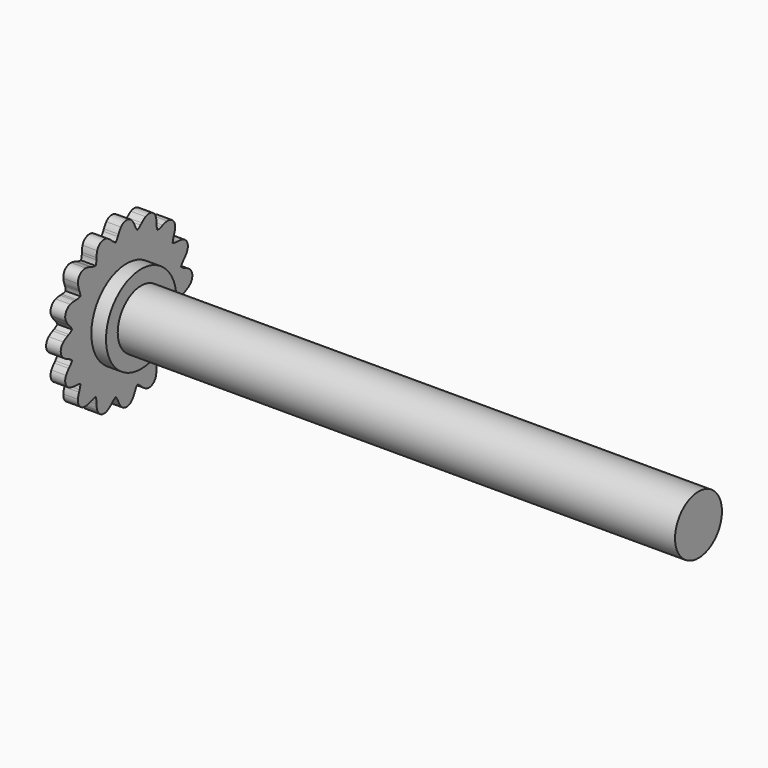
from build123d import *

# Parameters (mm, degrees)
F0_W     = 12.7
F0_H     = 12.7
F0_H_2   = 38.1
F2_R     = 25.4
F3_DEPTH = 508
F6_DEPTH = 508.001


# Not quite as in the source:
# - ends of sketch curves that miss each other by under 0.0002 mm in the source are joined


with BuildPart() as f1:
    # F0 (on Front) → F1 (revolve)
    with BuildSketch(Plane.XZ):
        with Locations((6.35, 31.75)):
            Rectangle(F0_W, F0_H)
        with Locations((19.05, 31.75)):
            Rectangle(F0_W, F0_H)
        with Locations((6.35, 57.15)):
            Rectangle(F0_W, F0_H_2)
        with Locations((19.05, -31.75)):
            Rectangle(F0_W, F0_H)
        with Locations((6.35, -31.75)):
            Rectangle(F0_W, F0_H)
        with Locations((6.35, -57.15)):
            Rectangle(F0_W, F0_H_2)
    revolve(axis=Axis((27.5155087221, 0, 0), (1, 0, 0)))


with BuildPart() as f3:
    # F2 (on face) → F3 (new body)
    with BuildSketch(Plane(origin=(0, 0, 0), x_dir=(0, -1, 0), z_dir=(-1, 0, 0))):
        Circle(F2_R)
    extrude(amount=-F3_DEPTH)

    # F4: union F1
    add(f1.part)

    # F5 (on face) → F6 (intersect, through all)
    with BuildSketch(Plane(origin=(0, 0, 0), x_dir=(0, -1, 0), z_dir=(-1, 0, 0))):
        with BuildLine():
            Line((9.3960515124, 62.4303196078), (8.6946709677, 63.9873266813))
            ThreePointArc((8.6946709677, 63.9873266813), (7.49940788, 66.2471696631), (6.0285111261, 68.338104117))
            ThreePointArc((6.0285111261, 68.338104117), (1.0289e-06, 71.2297171366), (-6.0285090682, 68.338104117))
            ThreePointArc((-6.0285090682, 68.338104117), (-7.4994058221, 66.2471696631), (-8.6946689099, 63.9873266813))
            Line((-8.6946689099, 63.9873266813), (-9.3960494545, 62.4303196078))
            ThreePointArc((-9.3960494545, 62.4303196078), (-10.4157598129, 60.5868350182), (-11.7228009421, 58.9345977067))
            ThreePointArc((-11.7228009421, 58.9345977067), (-13.5626685785, 59.9608761858), (-15.2102293125, 61.2738077372))
            Line((-15.2102293125, 61.2738077372), (-16.4540612533, 62.4438879902))
            ThreePointArc((-16.4540612533, 62.4438879902), (-18.4231448249, 64.0743032868), (-20.5822422039, 65.4431870141))
            ThreePointArc((-20.5822422039, 65.4431870141), (-27.2584316896, 65.8076781628), (-31.7214763845, 60.8291651421))
            ThreePointArc((-31.7214763845, 60.8291651421), (-32.2802418162, 58.3345057778), (-32.5197164501, 55.7892757193))
            Line((-32.5197164501, 55.7892757193), (-32.5718667687, 54.0823820379))
            ThreePointArc((-32.5718667687, 54.0823820379), (-32.8084852876, 51.9889980971), (-33.3837499896, 49.9623468766))
            ThreePointArc((-33.3837499896, 49.9623468766), (-35.4763058123, 50.2064176959), (-37.5008906056, 50.7889140871))
            Line((-37.5008906056, 50.7889140871), (-39.0978118049, 51.3939334078))
            ThreePointArc((-39.0978118049, 51.3939334078), (-41.5409407364, 52.14670507), (-44.0595357369, 52.5851379323))
            ThreePointArc((-44.0595357369, 52.5851379323), (-50.3670152817, 50.3670167368), (-52.5851364772, 44.059537192))
            ThreePointArc((-52.5851364772, 44.059537192), (-52.1467036149, 41.5409421915), (-51.3939319527, 39.09781326))
            Line((-51.3939319527, 39.09781326), (-50.788912632, 37.5008920607))
            ThreePointArc((-50.788912632, 37.5008920607), (-50.2064162869, 35.4763074971), (-49.9623257256, 33.3837816443))
            ThreePointArc((-49.9623257256, 33.3837816443), (-51.9889970797, 32.8084872341), (-54.0823812504, 32.5718686699))
            Line((-54.0823812504, 32.5718686699), (-55.7892749318, 32.5197183513))
            ThreePointArc((-55.7892749318, 32.5197183513), (-58.3345049903, 32.2802437174), (-60.8291643546, 31.7214782857))
            ThreePointArc((-60.8291643546, 31.7214782857), (-65.8076773753, 27.2584335908), (-65.4431862266, 20.5822441051))
            ThreePointArc((-65.4431862266, 20.5822441051), (-64.0743024993, 18.4231467261), (-62.4438872027, 16.4540631545))
            Line((-62.4438872027, 16.4540631545), (-61.2738069497, 15.2102312137))
            ThreePointArc((-61.2738069497, 15.2102312137), (-59.9608755289, 13.5626706742), (-58.9345902795, 11.7228382814))
            ThreePointArc((-58.9345902795, 11.7228382814), (-60.5868348232, 10.4157620005), (-62.4303196078, 9.3960515124))
            Line((-62.4303196078, 9.3960515124), (-63.9873266813, 8.6946709677))
            ThreePointArc((-63.9873266813, 8.6946709677), (-66.2471696631, 7.49940788), (-68.338104117, 6.0285111261))
            ThreePointArc((-68.338104117, 6.0285111261), (-71.2297171366, 1.0289e-06), (-68.338104117, -6.0285090682))
            ThreePointArc((-68.338104117, -6.0285090682), (-66.2471696631, -7.4994058221), (-63.9873266813, -8.6946689099))
            Line((-63.9873266813, -8.6946689099), (-62.4303196078, -9.3960494545))
            ThreePointArc((-62.4303196078, -9.3960494545), (-60.5868350182, -10.4157598129), (-58.9345977067, -11.7228009421))
            ThreePointArc((-58.9345977067, -11.7228009421), (-59.9608761858, -13.5626685785), (-61.2738077372, -15.2102293125))
            Line((-61.2738077372, -15.2102293125), (-62.4438879902, -16.4540612533))
            ThreePointArc((-62.4438879902, -16.4540612533), (-64.0743032868, -18.4231448249), (-65.4431870141, -20.5822422039))
            ThreePointArc((-65.4431870141, -20.5822422039), (-65.8076781628, -27.2584316896), (-60.8291651421, -31.7214763845))
            ThreePointArc((-60.8291651421, -31.7214763845), (-58.3345057778, -32.2802418162), (-55.7892757193, -32.5197164501))
            Line((-55.7892757193, -32.5197164501), (-54.0823820379, -32.5718667687))
            ThreePointArc((-54.0823820379, -32.5718667687), (-51.9889980971, -32.8084852876), (-49.9623468766, -33.3837499896))
            ThreePointArc((-49.9623468766, -33.3837499896), (-50.2064176959, -35.4763058123), (-50.7889140871, -37.5008906056))
            Line((-50.7889140871, -37.5008906056), (-51.3939334078, -39.0978118049))
            ThreePointArc((-51.3939334078, -39.0978118049), (-52.14670507, -41.5409407364), (-52.5851379323, -44.0595357369))
            ThreePointArc((-52.5851379323, -44.0595357369), (-50.3670167368, -50.3670152817), (-44.059537192, -52.5851364772))
            ThreePointArc((-44.059537192, -52.5851364772), (-41.5409421915, -52.1467036149), (-39.09781326, -51.3939319527))
            Line((-39.09781326, -51.3939319527), (-37.5008920607, -50.788912632))
            ThreePointArc((-37.5008920607, -50.788912632), (-35.4763074971, -50.2064162869), (-33.3837816443, -49.9623257256))
            ThreePointArc((-33.3837816443, -49.9623257256), (-32.8084872341, -51.9889970797), (-32.5718686699, -54.0823812504))
            Line((-32.5718686699, -54.0823812504), (-32.5197183513, -55.7892749318))
            ThreePointArc((-32.5197183513, -55.7892749318), (-32.2802437174, -58.3345049903), (-31.7214782857, -60.8291643546))
            ThreePointArc((-31.7214782857, -60.8291643546), (-27.2584335908, -65.8076773753), (-20.5822441051, -65.4431862266))
            ThreePointArc((-20.5822441051, -65.4431862266), (-18.4231467261, -64.0743024993), (-16.4540631545, -62.4438872027))
            Line((-16.4540631545, -62.4438872027), (-15.2102312137, -61.2738069497))
            ThreePointArc((-15.2102312137, -61.2738069497), (-13.5626706742, -59.9608755289), (-11.7228382814, -58.9345902795))
            ThreePointArc((-11.7228382814, -58.9345902795), (-10.4157620005, -60.5868348232), (-9.3960515124, -62.4303196078))
            Line((-9.3960515124, -62.4303196078), (-8.6946709677, -63.9873266813))
            ThreePointArc((-8.6946709677, -63.9873266813), (-7.49940788, -66.2471696631), (-6.0285111261, -68.338104117))
            ThreePointArc((-6.0285111261, -68.338104117), (-1.0289e-06, -71.2297171366), (6.0285090682, -68.338104117))
            ThreePointArc((6.0285090682, -68.338104117), (7.4994058221, -66.2471696631), (8.6946689099, -63.9873266813))
            Line((8.6946689099, -63.9873266813), (9.3960494545, -62.4303196078))
            ThreePointArc((9.3960494545, -62.4303196078), (10.4157598129, -60.5868350182), (11.7228009421, -58.9345977067))
            ThreePointArc((11.7228009421, -58.9345977067), (13.5626685785, -59.9608761858), (15.2102293125, -61.2738077372))
            Line((15.2102293125, -61.2738077372), (16.4540612533, -62.4438879902))
            ThreePointArc((16.4540612533, -62.4438879902), (18.4231448249, -64.0743032868), (20.5822422039, -65.4431870141))
            ThreePointArc((20.5822422039, -65.4431870141), (27.2584316896, -65.8076781628), (31.7214763845, -60.8291651421))
            ThreePointArc((31.7214763845, -60.8291651421), (32.2802418162, -58.3345057778), (32.5197164501, -55.7892757193))
            Line((32.5197164501, -55.7892757193), (32.5718667687, -54.0823820379))
            ThreePointArc((32.5718667687, -54.0823820379), (32.8084852876, -51.9889980971), (33.3837499896, -49.9623468766))
            ThreePointArc((33.3837499896, -49.9623468766), (35.4763058123, -50.2064176959), (37.5008906056, -50.7889140871))
            Line((37.5008906056, -50.7889140871), (39.0978118049, -51.3939334078))
            ThreePointArc((39.0978118049, -51.3939334078), (41.5409407364, -52.14670507), (44.0595357369, -52.5851379323))
            ThreePointArc((44.0595357369, -52.5851379323), (50.3670152817, -50.3670167368), (52.5851364772, -44.059537192))
            ThreePointArc((52.5851364772, -44.059537192), (52.1467036149, -41.5409421915), (51.3939319527, -39.09781326))
            Line((51.3939319527, -39.09781326), (50.788912632, -37.5008920607))
            ThreePointArc((50.788912632, -37.5008920607), (50.2064162869, -35.4763074971), (49.9623257256, -33.3837816443))
            ThreePointArc((49.9623257256, -33.3837816443), (51.9889970797, -32.8084872341), (54.0823812504, -32.5718686699))
            Line((54.0823812504, -32.5718686699), (55.7892749318, -32.5197183513))
            ThreePointArc((55.7892749318, -32.5197183513), (58.3345049903, -32.2802437174), (60.8291643546, -31.7214782857))
            ThreePointArc((60.8291643546, -31.7214782857), (65.8076773753, -27.2584335908), (65.4431862266, -20.5822441051))
            ThreePointArc((65.4431862266, -20.5822441051), (64.0743024993, -18.4231467261), (62.4438872027, -16.4540631545))
            Line((62.4438872027, -16.4540631545), (61.2738069497, -15.2102312137))
            ThreePointArc((61.2738069497, -15.2102312137), (59.9608755289, -13.5626706742), (58.9345902795, -11.7228382814))
            ThreePointArc((58.9345902795, -11.7228382814), (60.5868348232, -10.4157620005), (62.4303196078, -9.3960515124))
            Line((62.4303196078, -9.3960515124), (63.9873266813, -8.6946709677))
            ThreePointArc((63.9873266813, -8.6946709677), (66.2471696631, -7.49940788), (68.338104117, -6.0285111261))
            ThreePointArc((68.338104117, -6.0285111261), (71.2297171366, -1.0289e-06), (68.338104117, 6.0285090682))
            ThreePointArc((68.338104117, 6.0285090682), (66.2471696631, 7.4994058221), (63.9873266813, 8.6946689099))
            Line((63.9873266813, 8.6946689099), (62.4303196078, 9.3960494545))
            ThreePointArc((62.4303196078, 9.3960494545), (60.5868350182, 10.4157598129), (58.9345977067, 11.7228009421))
            ThreePointArc((58.9345977067, 11.7228009421), (59.9608761858, 13.5626685785), (61.2738077372, 15.2102293125))
            Line((61.2738077372, 15.2102293125), (62.4438879902, 16.4540612533))
            ThreePointArc((62.4438879902, 16.4540612533), (64.0743032868, 18.4231448249), (65.4431870141, 20.5822422039))
            ThreePointArc((65.4431870141, 20.5822422039), (65.8076781628, 27.2584316896), (60.8291651421, 31.7214763845))
            ThreePointArc((60.8291651421, 31.7214763845), (58.3345057778, 32.2802418162), (55.7892757193, 32.5197164501))
            Line((55.7892757193, 32.5197164501), (54.0823820379, 32.5718667687))
            ThreePointArc((54.0823820379, 32.5718667687), (51.9889980971, 32.8084852876), (49.9623468766, 33.3837499896))
            ThreePointArc((49.9623468766, 33.3837499896), (50.2064176959, 35.4763058123), (50.7889140871, 37.5008906056))
            Line((50.7889140871, 37.5008906056), (51.3939334078, 39.0978118049))
            ThreePointArc((51.3939334078, 39.0978118049), (52.14670507, 41.5409407364), (52.5851379323, 44.0595357369))
            ThreePointArc((52.5851379323, 44.0595357369), (50.3670167368, 50.3670152817), (44.059537192, 52.5851364772))
            ThreePointArc((44.059537192, 52.5851364772), (41.5409421915, 52.1467036149), (39.09781326, 51.3939319527))
            Line((39.09781326, 51.3939319527), (37.5008920607, 50.788912632))
            ThreePointArc((37.5008920607, 50.788912632), (35.4763074971, 50.2064162869), (33.3837816443, 49.9623257256))
            ThreePointArc((33.3837816443, 49.9623257256), (32.8084872341, 51.9889970797), (32.5718686699, 54.0823812504))
            Line((32.5718686699, 54.0823812504), (32.5197183513, 55.7892749318))
            ThreePointArc((32.5197183513, 55.7892749318), (32.2802437174, 58.3345049903), (31.7214782857, 60.8291643546))
            ThreePointArc((31.7214782857, 60.8291643546), (27.2584335908, 65.8076773753), (20.5822441051, 65.4431862266))
            ThreePointArc((20.5822441051, 65.4431862266), (18.4231467261, 64.0743024993), (16.4540631545, 62.4438872027))
            Line((16.4540631545, 62.4438872027), (15.2102312137, 61.2738069497))
            ThreePointArc((15.2102312137, 61.2738069497), (13.5626706742, 59.9608755289), (11.7228382814, 58.9345902795))
            ThreePointArc((11.7228382814, 58.9345902795), (10.4157620005, 60.5868348232), (9.3960515124, 62.4303196078))
        make_face()
    extrude(amount=-F6_DEPTH, mode=Mode.INTERSECT)


solid = f3.part
